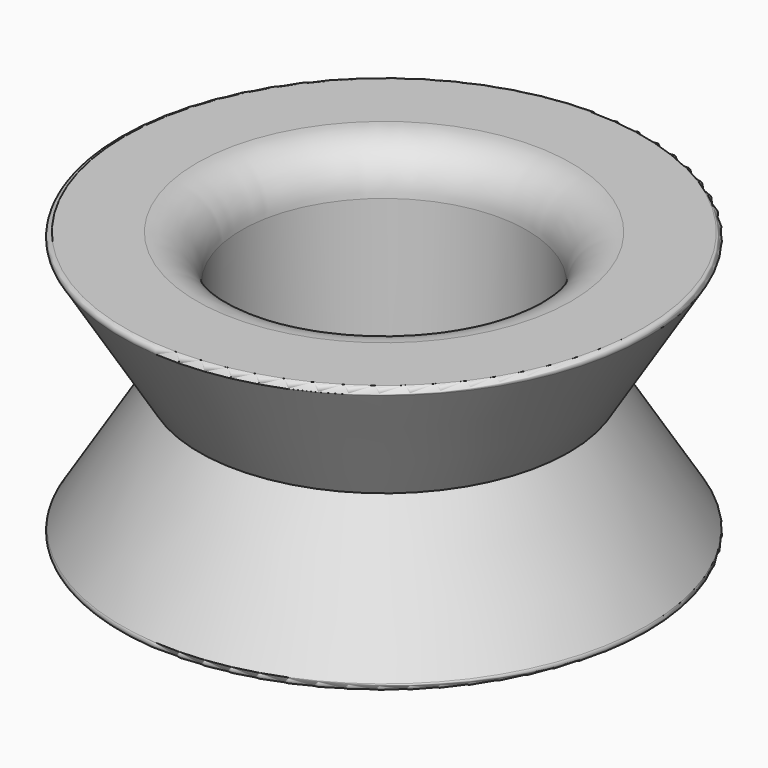
from build123d import *

# Parameters (mm, degrees)
F2_R = 0.5
F3_R = 0.05


with BuildPart() as f1:
    # F0 (on Front) → F1 (revolve)
    with BuildSketch(Plane.XZ):
        Polygon((1.6, 3), (1.6, 0), (3, 0), (2.0743638743, 1.5), (3, 3), align=None)
    revolve(axis=Axis((0, 0, 1.4736446901), (0, 0, -1)))

    # F2
    f2_edges = [f1.edges().sort_by_distance(p)[0] for p in [
        (-1.6, 0, 3),
        (-1.6, 0, 0),
    ]]
    fillet(f2_edges, radius=F2_R)

    # F3
    f3_edges = [f1.edges().sort_by_distance(p)[0] for p in [
        (-3, 0, 3),
        (-3, 0, 0),
    ]]
    fillet(f3_edges, radius=F3_R)


solid = f1.part
